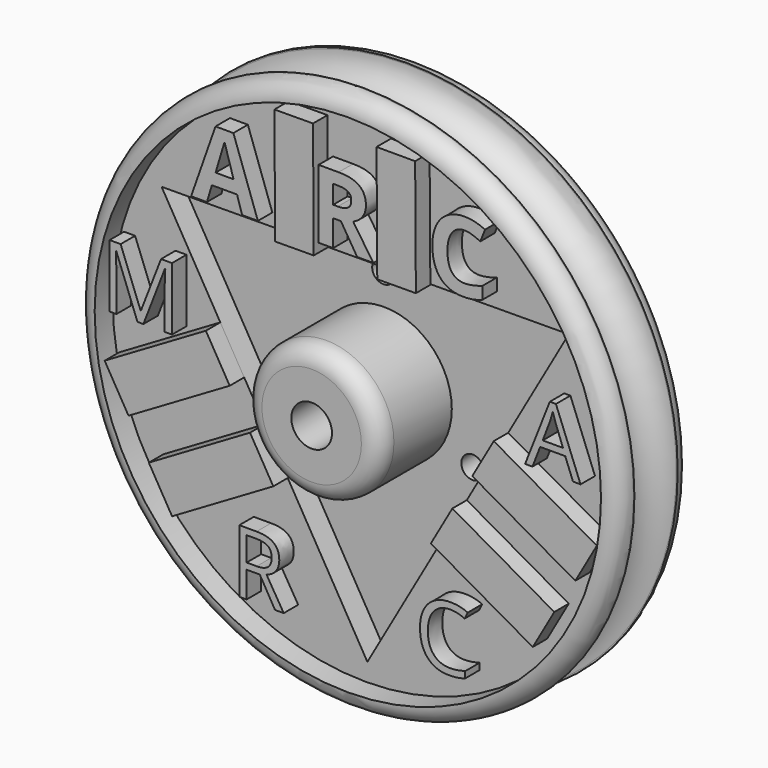
from build123d import *

# Parameters (mm, degrees)
F0_R            = 76.2
F1_DEPTH        = 25.4
F2_R            = 19.05
F3_DEPTH        = 12.7
F5_D            = 11.43
F6_R            = 5.08
F7_R            = 7.62
F9_DEPTH        = 6.35
F10_R           = 19.05
F11_DEPTH       = 6.35
F13_D           = 6.35
F15_DEPTH       = 5.08
F21_TEXT_SIZE   = 24.7832740166
F21_TEXT_SIZE_2 = 24.6099946206
F21_TEXT_SIZE_3 = 24.8002777778
F21_TEXT_SIZE_4 = 27.1816582729
F21_TEXT_SIZE_5 = 27.1991666667
F21_TEXT_SIZE_6 = 26.9765517241
F22_DEPTH       = 5.08


# Not quite as in the source:
# - the program builds the solid bodies; features that only make, move or delete a surface that nothing else refers to are left out
# - Text() gives the source's letters only with a copy of the font that has no kerning and outlines rounded to 1/6400 em; it was checked with that copy


with BuildPart() as f1:
    # F0 (on Front) → F1 (new body)
    with BuildSketch(Plane.XZ):
        Circle(F0_R)
    extrude(amount=F1_DEPTH)

    # F2 (on face) → F3 (join)
    with BuildSketch(Plane.XZ.offset(25.4)):
        Circle(F2_R)
    extrude(amount=F3_DEPTH)

    # F5 (through all)
    with Locations(Plane.XZ.offset(38.1)):
        with Locations((0, 0)):
            Hole(F5_D / 2)

    # F6
    f6_edges = [f1.edges().sort_by_distance(p)[0] for p in [
        (-76.2, -25.4, 0),
        (-19.05, -38.1, 0),
        (76.2, -12.7, 0),
        (-76.2, 0, 0),
    ]]
    fillet(f6_edges, radius=F6_R)

    # F7 (on Right) → F8 (revolve, cut)
    with BuildSketch(Plane.YZ):
        with Locations((-12.4054308981, 75.8084580302)):
            Circle(F7_R)
    revolve(axis=Axis((0, 0, 0), (0, 1, 0)), mode=Mode.SUBTRACT)

    # F9 (cut): a face of the model
    f9_faces = [f1.faces().sort_by_distance(p)[0] for p in [
        (-69.1084226289, -25.4, 0),
    ]]
    extrude(f9_faces, amount=-F9_DEPTH, mode=Mode.SUBTRACT)

    # F10 (on face) → F11 (cut)
    with BuildSketch(Plane.XZ.offset(19.05)):
        Polygon((0.4153364172, -66.0386939276), (56.9835183654, 33.3790388522), (-57.3988547826, 32.6596550754), align=None)
        Circle(F10_R, mode=Mode.SUBTRACT)
    extrude(amount=-F11_DEPTH, mode=Mode.SUBTRACT)

    # F13 (through all)
    with Locations(Plane.XZ.offset(12.7)):
        with Locations((-25.1830033958, -12.5195495784), (24.8951967806, -12.5195495784), (-0.1439040498, 27.773257345)):
            Hole(F13_D / 2)

    # F14 (on face) → F15 (join)
    with BuildSketch(Plane.XZ.offset(19.05)):
        Polygon((-21.6405968187, 65.4691243229), (-21.4356711209, 32.8858379231), (-10.5917977872, 32.9540381741), (-10.796723485, 65.5373245739), align=None)
        Polygon((17.8955433832, 65.5373245739), (7.0512411185, 65.5373245739), (7.2565957473, 32.8858379231), (18.100469081, 32.9540381741), align=None)
        Polygon((28.3497156943, -16.944440609), (22.3041939704, -27.5693545192), (50.9379966416, -43.8618419264), (56.9835183654, -33.2369280163), align=None)
        Polygon((39.9815774634, 3.4983822866), (33.9395412745, -7.1204058482), (62.8862345329, -23.5909264007), (68.9282707218, -12.9721382659), align=None)
        Polygon((-62.6287566209, -23.5909264007), (-34.2027476517, -6.9399212502), (-40.8971556101, 4.4885360081), (-69.3231645794, -12.1624691424), align=None)
        Polygon((-21.9614577056, -27.8378198849), (-28.4917591827, -16.6895194261), (-56.9177681519, -33.3405245766), (-50.3874666748, -44.4888250354), align=None)
    extrude(amount=F15_DEPTH)

    # F21 (on face) → F22 (join)
    with BuildSketch(Plane.XZ.offset(19.05)):
        with Locations((-70.3685060143, 0.43170969)):
            Text('M', F21_TEXT_SIZE, font='Open Sans', text_align=(TextAlign.LEFT, TextAlign.BOTTOM))
        with Locations((48.7830713391, 0.7195144426)):
            Text('A', F21_TEXT_SIZE_2, font='Open Sans', text_align=(TextAlign.LEFT, TextAlign.BOTTOM))
        with Locations((-33.9343240409, -58.2405565701)):
            Text('R', F21_TEXT_SIZE_3, font='Open Sans', text_align=(TextAlign.LEFT, TextAlign.BOTTOM))
        with Locations((17.7454914862, -58.2405565701)):
            Text('C', F21_TEXT_SIZE_3, font='Open Sans', text_align=(TextAlign.LEFT, TextAlign.BOTTOM))
        with Locations((-45.0416021049, 36.4074259996)):
            Text('A', F21_TEXT_SIZE_4, font='Open Sans', font_style=FontStyle.BOLD, text_align=(TextAlign.LEFT, TextAlign.BOTTOM))
        with Locations((21.1505375079, 36.6734343831)):
            Text('C', F21_TEXT_SIZE_5, font='Open Sans', font_style=FontStyle.BOLD, text_align=(TextAlign.LEFT, TextAlign.BOTTOM))
        with Locations((-11.6561349278, 36.5551027148)):
            Text('R', F21_TEXT_SIZE_6, font='Open Sans', font_style=FontStyle.BOLD, text_align=(TextAlign.LEFT, TextAlign.BOTTOM))
    extrude(amount=F22_DEPTH)


solid = f1.part
